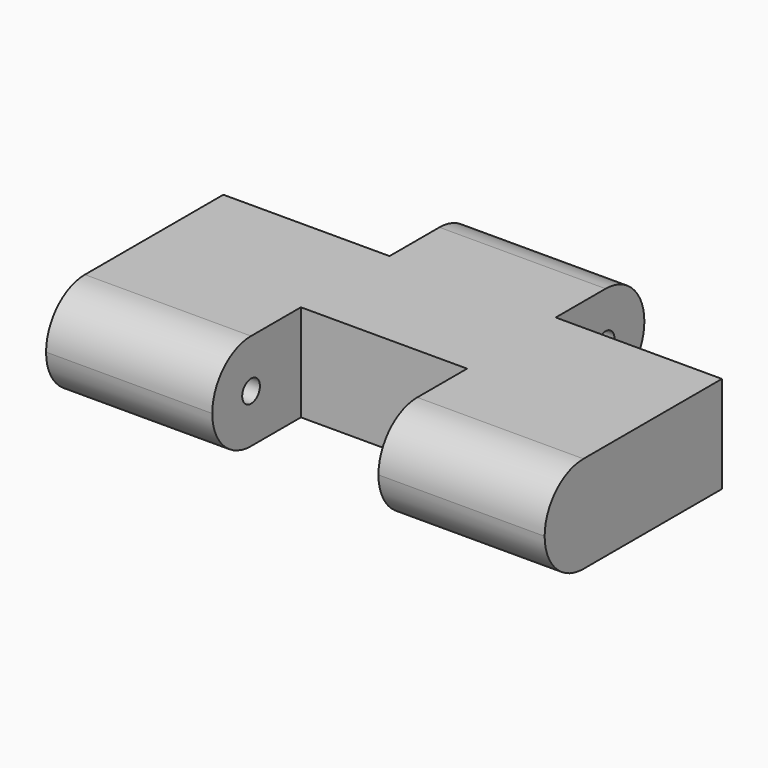
from build123d import *

# Parameters (mm, degrees)
F1_DEPTH = 22.225
F2_R     = 22.22499
F3_R     = 5.08
F4_DEPTH = 114.301
F5_DEPTH = 114.301
F6_R     = 5.08
F7_DEPTH = 63.5


# Not quite as in the source:
# - a fillet or chamfer is up to 0.001 mm smaller than in the source, because OpenCascade refuses the exact size


with BuildPart() as f1:
    # F0 (on Top) → F1 (new body, symmetric)
    with BuildSketch(Plane.XY):
        Polygon((38.1, 40.6722736142), (0, 40.6722736142), (-38.1, 40.6722736142), (-38.1, -10.1277263858), (-114.3, -10.1277263858), (-114.3, -111.7277263858), (-38.1, -111.7277263858), (-38.1, -60.9277263858), (38.1, -60.9277263858), (38.1, -111.7277263858), (114.3, -111.7277263858), (114.3, -10.1277263858), (38.1, -10.1277263858), align=None)
    extrude(amount=F1_DEPTH, both=True)

    # F2 (radius 22.225 in the source; OpenCascade refuses exactly that, so slightly less here)
    f2_edges = [f1.edges().sort_by_distance(p)[0] for p in [
        (-76.2, -111.727726, 22.225),
        (-76.2, -111.727726, -22.225),
        (76.2, -111.727726, 22.225),
        (76.2, -111.727726, -22.225),
        (0, 40.672274, 22.225),
        (0, 40.672274, -22.225),
    ]]
    fillet(f2_edges, radius=F2_R)

    # F3 (on Right) → F4 (cut, through all)
    with BuildSketch(Plane.YZ):
        with Locations((18.4472736142, 0)):
            Circle(F3_R)
    extrude(amount=-F4_DEPTH, mode=Mode.SUBTRACT)

    # F3 (on Right) → F5 (cut, through all)
    with BuildSketch(Plane.YZ):
        with Locations((18.4472736142, 0)):
            Circle(F3_R)
    extrude(amount=F5_DEPTH, mode=Mode.SUBTRACT)

    # F6 (on Right) → F7 (cut, symmetric)
    with BuildSketch(Plane.YZ):
        with Locations((-89.5027263858, 0)):
            Circle(F6_R)
    extrude(amount=F7_DEPTH, both=True, mode=Mode.SUBTRACT)


solid = f1.part
